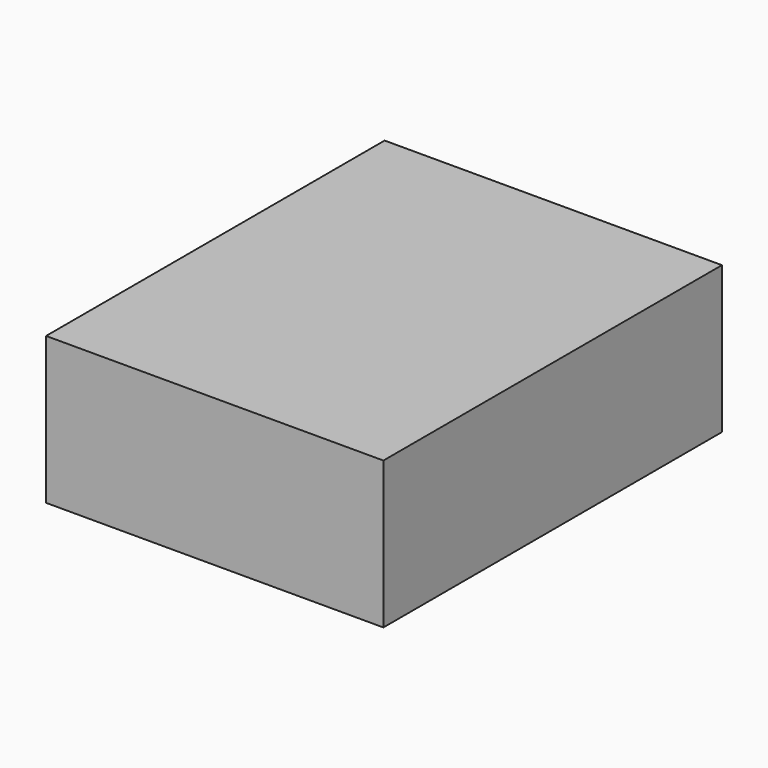
from build123d import *

# Parameters (mm, degrees)
F1_W     = 69.3769939244
F1_H     = 87.0304815471
F2_DEPTH = 30.226


# Not quite as in the source:
# - a feature of the source that left no trace in its solid (it failed there, or was rolled back) is left out


with BuildPart() as f2:
    # F1 (on face) → F2 (new body)
    with BuildSketch(Plane.XY):
        with Locations((-0.8827243, 0.582812354)):
            Rectangle(F1_W, F1_H)
    extrude(amount=F2_DEPTH)


solid = f2.part
